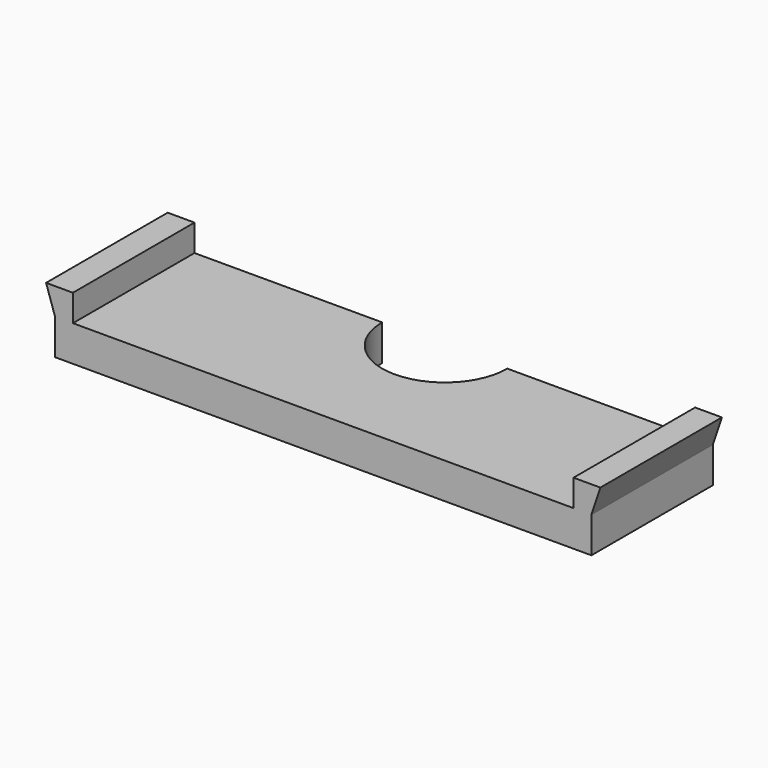
from build123d import *

# Parameters (mm, degrees)
F0_W     = 76.2
F0_H     = 21.59
F1_DEPTH = 5.08
F2_W     = 2.54
F2_H     = 21.59
F3_DEPTH = 3.81
F5_DEPTH = 25.4
F7_DEPTH = 21.59


# Not quite as in the source:
# - a feature names something its author has since deleted; it is built from what else it names


with BuildPart() as f1:
    # F0 (on Top) → F1 (new body)
    with BuildSketch(Plane.XY):
        with Locations((38.1, 10.795)):
            Rectangle(F0_W, F0_H)
    extrude(amount=F1_DEPTH)

    # F2 (on face) → F3 (join)
    with BuildSketch(Plane.XY.offset(5.08)):
        with Locations((1.27, 10.795)):
            Rectangle(F2_W, F2_H)
        with Locations((74.93, 10.795)):
            Rectangle(F2_W, F2_H)
    extrude(amount=F3_DEPTH)

    # F4 (on face) → F5 (cut)
    with BuildSketch(Plane.XY.offset(5.08)):
        with BuildLine():
            ThreePointArc((29.21, 21.59), (38.1, 12.7), (46.99, 21.59))
            Line((46.99, 21.59), (29.21, 21.59))
        make_face()
        with BuildLine():
            Line((29.21, 21.59), (46.99, 21.59))
            ThreePointArc((46.99, 21.59), (38.1, 30.48), (29.21, 21.59))
        make_face()
    extrude(amount=-F5_DEPTH, mode=Mode.SUBTRACT)

    # F6 (on face) → F7 (join, through all)
    with BuildSketch(Plane.XZ):
        Polygon((0, 5.08), (0, 8.89), (-1.27, 8.89), align=None)
        Polygon((76.2, 8.89), (76.2, 5.08), (77.47, 8.89), align=None)
    extrude(amount=-F7_DEPTH)


solid = f1.part
